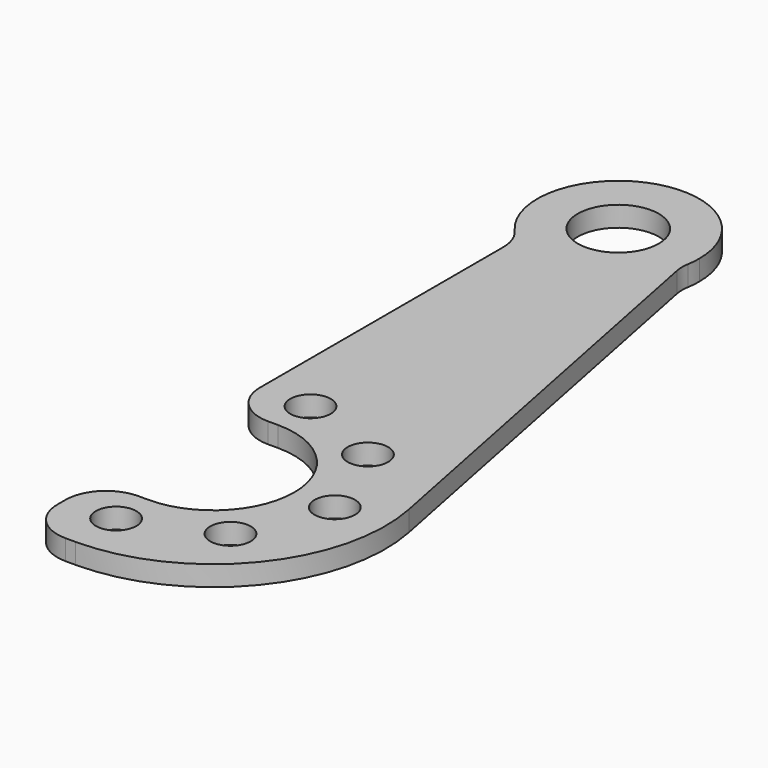
from build123d import *

# Parameters (mm, degrees)
F0_R     = 1
F0_R_2   = 2
F1_DEPTH = 1
F2_R     = 2


with BuildPart() as f1:
    # F0 (on Top) → F1 (new body)
    with BuildSketch(Plane.XY):
        with BuildLine():
            ThreePointArc((-2.5, 28.1224989992), (-4, 25), (-2.5, 21.8775010008))
            Line((-2.5, 21.8775010008), (-2.5, 28.1224989992))
        make_face()
        with BuildLine():
            ThreePointArc((1.9364916731, 28.5), (0, 29), (-1.9364916731, 28.5))
            Line((-1.9364916731, 28.5), (1.9364916731, 28.5))
        make_face()
        with BuildLine():
            Line((3.2255519271, 27.3655474558), (3.8851082618, 24.0481944557))
            ThreePointArc((3.8851082618, 24.0481944557), (3.9711731923, 24.5206426422), (4, 25))
            ThreePointArc((4, 25), (3.8014607527, 26.2445465624), (3.2255519271, 27.3655474558))
        make_face()
        with BuildLine():
            ThreePointArc((0, -8.5), (-1.2640556872, -8.4054841157), (-2.5, -8.1240384046))
            Line((-2.5, -8.1240384046), (-2.5, -8.5))
            Line((-2.5, -8.5), (0, -8.5))
        make_face()
        with BuildLine():
            ThreePointArc((0, 4), (4, 0), (0, -4))
            Line((0, -4), (-2.5, -4))
            Line((-2.5, -4), (-2.5, -8.1240384046))
            ThreePointArc((-2.5, -8.1240384046), (-1.2640556872, -8.4054841157), (0, -8.5))
            ThreePointArc((0, -8.5), (6.5703494482, -5.3926346185), (8.3368220918, 1.6575274991))
            Line((8.3368220918, 1.6575274991), (3.8851082618, 24.0481944557))
            ThreePointArc((3.8851082618, 24.0481944557), (1.2874815505, 21.2128650332), (-2.5, 21.8775010008))
            Line((-2.5, 21.8775010008), (-2.5, 4))
            Line((-2.5, 4), (0, 4))
        make_face()
        with Locations((0, -6)):
            Circle(F0_R, mode=Mode.SUBTRACT)
        with Locations((0, 6)):
            Circle(F0_R, mode=Mode.SUBTRACT)
        with Locations((4.2426406871, -4.2426406871)):
            Circle(F0_R, mode=Mode.SUBTRACT)
        with Locations((6, 0)):
            Circle(F0_R, mode=Mode.SUBTRACT)
        with Locations((4.2426406871, 4.2426406871)):
            Circle(F0_R, mode=Mode.SUBTRACT)
        with BuildLine():
            Line((-2.5, 28.1224989992), (-2.5, 21.8775010008))
            ThreePointArc((-2.5, 21.8775010008), (1.2874815505, 21.2128650332), (3.8851082618, 24.0481944557))
            Line((3.8851082618, 24.0481944557), (3.2255519271, 27.3655474558))
            ThreePointArc((3.2255519271, 27.3655474558), (2.6426159721, 28.002762199), (1.9364916731, 28.5))
            Line((1.9364916731, 28.5), (-1.9364916731, 28.5))
            ThreePointArc((-1.9364916731, 28.5), (-2.2262617418, 28.3232151085), (-2.5, 28.1224989992))
        make_face()
        with Locations((0, 25)):
            Circle(F0_R_2, mode=Mode.SUBTRACT)
    extrude(amount=F1_DEPTH)

    # F2
    f2_edges = [f1.edges().sort_by_distance(p)[0] for p in [
        (-2.5, 4, 0.5),
        (-2.5, -4, 0.5),
        (-2.5, -8.5, 0.5),
        (-2.5, 21.877501, 0.5),
        (3.885108, 24.048194, 0.5),
    ]]
    fillet(f2_edges, radius=F2_R)


solid = f1.part
